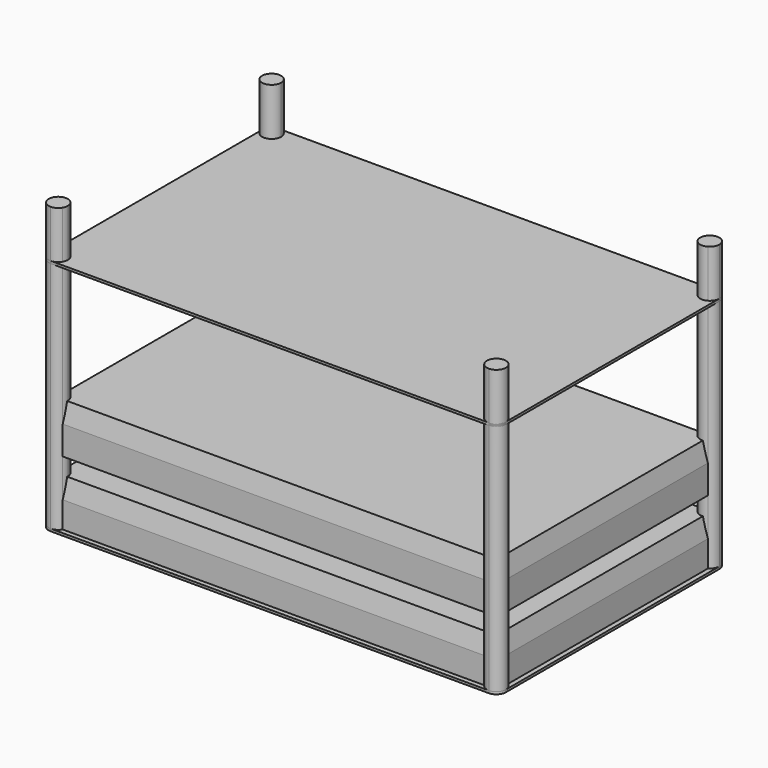
from build123d import *

# Parameters (mm, degrees)
F1_DEPTH = 6.35
F2_START = 6.35
F2_DEPTH = 120.65
F3_SIZE2 = 10.7978733328
F3_SIZE  = 50.8
F4_START = 6.35
F4_DEPTH = 755.65
F5_START = 628.65
F5_DEPTH = 6.35
F6_START = 177.8
F6_DEPTH = 127
F7_SIZE2 = 10.7978733328
F7_SIZE  = 50.8


# Not quite as in the source:
# - a feature names something its author has since deleted; it is built from what else it names


with BuildPart() as f1:
    # F0 (on Top) → F1 (new body)
    with BuildSketch(Plane.XY):
        Polygon((-421.6065403938, 372.1638967734), (-535.9065403938, 372.1638967734), (-535.9065403938, -364.4361032266), (-421.6065403938, -364.4361032266), (-383.5065403938, -364.4361032266), (378.4934596062, -364.4361032266), (416.5934596062, -364.4361032266), (530.8934596062, -364.4361032266), (530.8934596062, -219.4858193398), (530.8934596062, 237.7141806602), (530.8934596062, 372.1638967734), (416.5934596062, 372.1638967734), (378.4934596062, 372.1638967734), (-383.5065403938, 372.1638967734), align=None)
        Polygon((530.8934596062, 384.8638967734), (-535.9065403938, 384.8638967734), (-535.9065403938, 372.1638967734), (-421.6065403938, 372.1638967734), (-383.5065403938, 372.1638967734), (378.4934596062, 372.1638967734), (416.5934596062, 372.1638967734), (530.8934596062, 372.1638967734), align=None)
        Polygon((-421.6065403938, -364.4361032266), (-535.9065403938, -364.4361032266), (-535.9065403938, -377.1361032266), (530.8934596062, -377.1361032266), (530.8934596062, -364.4361032266), (416.5934596062, -364.4361032266), (378.4934596062, -364.4361032266), (-383.5065403938, -364.4361032266), align=None)
        with BuildLine():
            Line((607.0934596062, -351.7361032266), (607.0934596062, 359.4638967734))
            ThreePointArc((607.0934596062, 359.4638967734), (603.6905048623, 346.7638967734), (594.3934596062, 337.4668515172))
            Line((594.3934596062, 337.4668515172), (594.3934596062, 22.9138967734))
            Line((594.3934596062, 22.9138967734), (594.3934596062, -15.1861032266))
            Line((594.3934596062, -15.1861032266), (594.3934596062, -329.7390579705))
            ThreePointArc((594.3934596062, -329.7390579705), (603.6905048623, -339.0361032266), (607.0934596062, -351.7361032266))
        make_face()
        with BuildLine():
            ThreePointArc((-599.4065403938, 337.4668515172), (-608.70358565, 346.7638967734), (-612.1065403938, 359.4638967734))
            Line((-612.1065403938, 359.4638967734), (-612.1065403938, -351.7361032266))
            ThreePointArc((-612.1065403938, -351.7361032266), (-608.70358565, -339.0361032266), (-599.4065403938, -329.7390579705))
            Line((-599.4065403938, -329.7390579705), (-599.4065403938, -15.1861032266))
            Line((-599.4065403938, -15.1861032266), (-599.4065403938, 22.9138967734))
            Line((-599.4065403938, 22.9138967734), (-599.4065403938, 337.4668515172))
        make_face()
        with BuildLine():
            ThreePointArc((-561.3065403938, 359.4638967734), (-562.1720244061, 366.037900519), (-564.7094951377, 372.1638967734))
            Line((-564.7094951377, 372.1638967734), (-586.7065403938, 372.1638967734))
            ThreePointArc((-586.7065403938, 372.1638967734), (-595.6867965149, 368.4441528944), (-599.4065403938, 359.4638967734))
            Line((-599.4065403938, 359.4638967734), (-599.4065403938, 337.4668515172))
            ThreePointArc((-599.4065403938, 337.4668515172), (-574.0065403938, 337.4668515172), (-561.3065403938, 359.4638967734))
        make_face()
        with BuildLine():
            Line((581.6934596062, 372.1638967734), (559.69641435, 372.1638967734))
            ThreePointArc((559.69641435, 372.1638967734), (563.732947364, 341.5033845312), (594.3934596062, 337.4668515172))
            Line((594.3934596062, 337.4668515172), (594.3934596062, 359.4638967734))
            ThreePointArc((594.3934596062, 359.4638967734), (590.6737157272, 368.4441528944), (581.6934596062, 372.1638967734))
        make_face()
        with BuildLine():
            ThreePointArc((-561.3065403938, -351.7361032266), (-574.0065403938, -329.7390579705), (-599.4065403938, -329.7390579705))
            Line((-599.4065403938, -329.7390579705), (-599.4065403938, -351.7361032266))
            ThreePointArc((-599.4065403938, -351.7361032266), (-595.6867965149, -360.7163593477), (-586.7065403938, -364.4361032266))
            Line((-586.7065403938, -364.4361032266), (-564.7094951377, -364.4361032266))
            ThreePointArc((-564.7094951377, -364.4361032266), (-562.1720244061, -358.3101069722), (-561.3065403938, -351.7361032266))
        make_face()
        with BuildLine():
            Line((-535.9065403938, 372.1638967734), (-564.7094951377, 372.1638967734))
            ThreePointArc((-564.7094951377, 372.1638967734), (-562.1720244061, 366.037900519), (-561.3065403938, 359.4638967734))
            ThreePointArc((-561.3065403938, 359.4638967734), (-574.0065403938, 337.4668515172), (-599.4065403938, 337.4668515172))
            Line((-599.4065403938, 337.4668515172), (-599.4065403938, 22.9138967734))
            Line((-599.4065403938, 22.9138967734), (-599.4065403938, -15.1861032266))
            Line((-599.4065403938, -15.1861032266), (-599.4065403938, -329.7390579705))
            ThreePointArc((-599.4065403938, -329.7390579705), (-574.0065403938, -329.7390579705), (-561.3065403938, -351.7361032266))
            ThreePointArc((-561.3065403938, -351.7361032266), (-562.1720244061, -358.3101069722), (-564.7094951377, -364.4361032266))
            Line((-564.7094951377, -364.4361032266), (-535.9065403938, -364.4361032266))
            Line((-535.9065403938, -364.4361032266), (-535.9065403938, 372.1638967734))
        make_face()
        with BuildLine():
            Line((594.3934596062, -351.7361032266), (594.3934596062, -329.7390579705))
            ThreePointArc((594.3934596062, -329.7390579705), (563.732947364, -333.7755909845), (559.69641435, -364.4361032266))
            Line((559.69641435, -364.4361032266), (581.6934596062, -364.4361032266))
            ThreePointArc((581.6934596062, -364.4361032266), (590.6737157272, -360.7163593477), (594.3934596062, -351.7361032266))
        make_face()
        with BuildLine():
            Line((559.69641435, 372.1638967734), (530.8934596062, 372.1638967734))
            Line((530.8934596062, 372.1638967734), (530.8934596062, 237.7141806602))
            Line((530.8934596062, 237.7141806602), (530.8934596062, -219.4858193398))
            Line((530.8934596062, -219.4858193398), (530.8934596062, -364.4361032266))
            Line((530.8934596062, -364.4361032266), (559.69641435, -364.4361032266))
            ThreePointArc((559.69641435, -364.4361032266), (563.732947364, -333.7755909845), (594.3934596062, -329.7390579705))
            Line((594.3934596062, -329.7390579705), (594.3934596062, -15.1861032266))
            Line((594.3934596062, -15.1861032266), (594.3934596062, 22.9138967734))
            Line((594.3934596062, 22.9138967734), (594.3934596062, 337.4668515172))
            ThreePointArc((594.3934596062, 337.4668515172), (563.732947364, 341.5033845312), (559.69641435, 372.1638967734))
        make_face()
        with BuildLine():
            ThreePointArc((581.6934596062, -377.1361032266), (599.6539718483, -369.6966154688), (607.0934596062, -351.7361032266))
            ThreePointArc((607.0934596062, -351.7361032266), (603.6905048623, -339.0361032266), (594.3934596062, -329.7390579705))
            Line((594.3934596062, -329.7390579705), (594.3934596062, -351.7361032266))
            ThreePointArc((594.3934596062, -351.7361032266), (590.6737157272, -360.7163593477), (581.6934596062, -364.4361032266))
            Line((581.6934596062, -364.4361032266), (559.69641435, -364.4361032266))
            ThreePointArc((559.69641435, -364.4361032266), (568.9934596062, -373.7331484828), (581.6934596062, -377.1361032266))
        make_face()
        with BuildLine():
            Line((530.8934596062, -364.4361032266), (530.8934596062, -377.1361032266))
            Line((530.8934596062, -377.1361032266), (581.6934596062, -377.1361032266))
            ThreePointArc((581.6934596062, -377.1361032266), (568.9934596062, -373.7331484828), (559.69641435, -364.4361032266))
            Line((559.69641435, -364.4361032266), (530.8934596062, -364.4361032266))
        make_face()
        with BuildLine():
            ThreePointArc((607.0934596062, 359.4638967734), (599.6539718483, 377.4244090155), (581.6934596062, 384.8638967734))
            ThreePointArc((581.6934596062, 384.8638967734), (568.9934596062, 381.4609420295), (559.69641435, 372.1638967734))
            Line((559.69641435, 372.1638967734), (581.6934596062, 372.1638967734))
            ThreePointArc((581.6934596062, 372.1638967734), (590.6737157272, 368.4441528944), (594.3934596062, 359.4638967734))
            Line((594.3934596062, 359.4638967734), (594.3934596062, 337.4668515172))
            ThreePointArc((594.3934596062, 337.4668515172), (603.6905048623, 346.7638967734), (607.0934596062, 359.4638967734))
        make_face()
        with BuildLine():
            Line((581.6934596062, 384.8638967734), (530.8934596062, 384.8638967734))
            Line((530.8934596062, 384.8638967734), (530.8934596062, 372.1638967734))
            Line((530.8934596062, 372.1638967734), (559.69641435, 372.1638967734))
            ThreePointArc((559.69641435, 372.1638967734), (568.9934596062, 381.4609420295), (581.6934596062, 384.8638967734))
        make_face()
        with BuildLine():
            Line((-535.9065403938, -377.1361032266), (-535.9065403938, -364.4361032266))
            Line((-535.9065403938, -364.4361032266), (-564.7094951377, -364.4361032266))
            ThreePointArc((-564.7094951377, -364.4361032266), (-574.0065403938, -373.7331484828), (-586.7065403938, -377.1361032266))
            Line((-586.7065403938, -377.1361032266), (-535.9065403938, -377.1361032266))
        make_face()
        with BuildLine():
            ThreePointArc((-599.4065403938, -329.7390579705), (-608.70358565, -339.0361032266), (-612.1065403938, -351.7361032266))
            ThreePointArc((-612.1065403938, -351.7361032266), (-604.667052636, -369.6966154688), (-586.7065403938, -377.1361032266))
            ThreePointArc((-586.7065403938, -377.1361032266), (-574.0065403938, -373.7331484828), (-564.7094951377, -364.4361032266))
            Line((-564.7094951377, -364.4361032266), (-586.7065403938, -364.4361032266))
            ThreePointArc((-586.7065403938, -364.4361032266), (-595.6867965149, -360.7163593477), (-599.4065403938, -351.7361032266))
            Line((-599.4065403938, -351.7361032266), (-599.4065403938, -329.7390579705))
        make_face()
        with BuildLine():
            Line((-535.9065403938, 384.8638967734), (-586.7065403938, 384.8638967734))
            ThreePointArc((-586.7065403938, 384.8638967734), (-574.0065403938, 381.4609420295), (-564.7094951377, 372.1638967734))
            Line((-564.7094951377, 372.1638967734), (-535.9065403938, 372.1638967734))
            Line((-535.9065403938, 372.1638967734), (-535.9065403938, 384.8638967734))
        make_face()
        with BuildLine():
            ThreePointArc((-564.7094951377, 372.1638967734), (-574.0065403938, 381.4609420295), (-586.7065403938, 384.8638967734))
            ThreePointArc((-586.7065403938, 384.8638967734), (-604.667052636, 377.4244090155), (-612.1065403938, 359.4638967734))
            ThreePointArc((-612.1065403938, 359.4638967734), (-608.70358565, 346.7638967734), (-599.4065403938, 337.4668515172))
            Line((-599.4065403938, 337.4668515172), (-599.4065403938, 359.4638967734))
            ThreePointArc((-599.4065403938, 359.4638967734), (-595.6867965149, 368.4441528944), (-586.7065403938, 372.1638967734))
            Line((-586.7065403938, 372.1638967734), (-564.7094951377, 372.1638967734))
        make_face()
    extrude(amount=F1_DEPTH)


with BuildPart() as f2:
    # F0 (on Top) → F2 (new body)
    with BuildSketch(Plane.XY.offset(F2_START)):
        Polygon((-421.6065403938, 372.1638967734), (-535.9065403938, 372.1638967734), (-535.9065403938, -364.4361032266), (-421.6065403938, -364.4361032266), (-383.5065403938, -364.4361032266), (378.4934596062, -364.4361032266), (416.5934596062, -364.4361032266), (530.8934596062, -364.4361032266), (530.8934596062, -219.4858193398), (530.8934596062, 237.7141806602), (530.8934596062, 372.1638967734), (416.5934596062, 372.1638967734), (378.4934596062, 372.1638967734), (-383.5065403938, 372.1638967734), align=None)
        with BuildLine():
            Line((-535.9065403938, 372.1638967734), (-564.7094951377, 372.1638967734))
            ThreePointArc((-564.7094951377, 372.1638967734), (-562.1720244061, 366.037900519), (-561.3065403938, 359.4638967734))
            ThreePointArc((-561.3065403938, 359.4638967734), (-574.0065403938, 337.4668515172), (-599.4065403938, 337.4668515172))
            Line((-599.4065403938, 337.4668515172), (-599.4065403938, 22.9138967734))
            Line((-599.4065403938, 22.9138967734), (-599.4065403938, -15.1861032266))
            Line((-599.4065403938, -15.1861032266), (-599.4065403938, -329.7390579705))
            ThreePointArc((-599.4065403938, -329.7390579705), (-574.0065403938, -329.7390579705), (-561.3065403938, -351.7361032266))
            ThreePointArc((-561.3065403938, -351.7361032266), (-562.1720244061, -358.3101069722), (-564.7094951377, -364.4361032266))
            Line((-564.7094951377, -364.4361032266), (-535.9065403938, -364.4361032266))
            Line((-535.9065403938, -364.4361032266), (-535.9065403938, 372.1638967734))
        make_face()
        with BuildLine():
            Line((559.69641435, 372.1638967734), (530.8934596062, 372.1638967734))
            Line((530.8934596062, 372.1638967734), (530.8934596062, 237.7141806602))
            Line((530.8934596062, 237.7141806602), (530.8934596062, -219.4858193398))
            Line((530.8934596062, -219.4858193398), (530.8934596062, -364.4361032266))
            Line((530.8934596062, -364.4361032266), (559.69641435, -364.4361032266))
            ThreePointArc((559.69641435, -364.4361032266), (563.732947364, -333.7755909845), (594.3934596062, -329.7390579705))
            Line((594.3934596062, -329.7390579705), (594.3934596062, -15.1861032266))
            Line((594.3934596062, -15.1861032266), (594.3934596062, 22.9138967734))
            Line((594.3934596062, 22.9138967734), (594.3934596062, 337.4668515172))
            ThreePointArc((594.3934596062, 337.4668515172), (563.732947364, 341.5033845312), (559.69641435, 372.1638967734))
        make_face()
        with BuildLine():
            ThreePointArc((-561.3065403938, 359.4638967734), (-562.1720244061, 366.037900519), (-564.7094951377, 372.1638967734))
            Line((-564.7094951377, 372.1638967734), (-586.7065403938, 372.1638967734))
            ThreePointArc((-586.7065403938, 372.1638967734), (-595.6867965149, 368.4441528944), (-599.4065403938, 359.4638967734))
            Line((-599.4065403938, 359.4638967734), (-599.4065403938, 337.4668515172))
            ThreePointArc((-599.4065403938, 337.4668515172), (-574.0065403938, 337.4668515172), (-561.3065403938, 359.4638967734))
        make_face()
        with BuildLine():
            Line((581.6934596062, 372.1638967734), (559.69641435, 372.1638967734))
            ThreePointArc((559.69641435, 372.1638967734), (563.732947364, 341.5033845312), (594.3934596062, 337.4668515172))
            Line((594.3934596062, 337.4668515172), (594.3934596062, 359.4638967734))
            ThreePointArc((594.3934596062, 359.4638967734), (590.6737157272, 368.4441528944), (581.6934596062, 372.1638967734))
        make_face()
        with BuildLine():
            ThreePointArc((-561.3065403938, -351.7361032266), (-574.0065403938, -329.7390579705), (-599.4065403938, -329.7390579705))
            Line((-599.4065403938, -329.7390579705), (-599.4065403938, -351.7361032266))
            ThreePointArc((-599.4065403938, -351.7361032266), (-595.6867965149, -360.7163593477), (-586.7065403938, -364.4361032266))
            Line((-586.7065403938, -364.4361032266), (-564.7094951377, -364.4361032266))
            ThreePointArc((-564.7094951377, -364.4361032266), (-562.1720244061, -358.3101069722), (-561.3065403938, -351.7361032266))
        make_face()
        with BuildLine():
            Line((594.3934596062, -351.7361032266), (594.3934596062, -329.7390579705))
            ThreePointArc((594.3934596062, -329.7390579705), (563.732947364, -333.7755909845), (559.69641435, -364.4361032266))
            Line((559.69641435, -364.4361032266), (581.6934596062, -364.4361032266))
            ThreePointArc((581.6934596062, -364.4361032266), (590.6737157272, -360.7163593477), (594.3934596062, -351.7361032266))
        make_face()
    extrude(amount=F2_DEPTH)

    # F3
    f3_edges = [f2.edges().sort_by_distance(p)[0] for p in [
        (590.673716, 368.444153, 127),
        (-2.50654, 372.163897, 127),
        (-595.686797, 368.444153, 127),
        (-599.40654, 3.863897, 127),
        (-595.686797, -360.716359, 127),
        (-2.50654, -364.436103, 127),
        (590.673716, -360.716359, 127),
        (594.39346, 3.863897, 127),
    ]]
    chamfer(f3_edges, length=F3_SIZE, length2=F3_SIZE2)


with BuildPart() as f4:
    # F0 (on Top) → F4 (new body)
    with BuildSketch(Plane.XY.offset(F4_START)):
        with BuildLine():
            ThreePointArc((581.6934596062, -377.1361032266), (599.6539718483, -369.6966154688), (607.0934596062, -351.7361032266))
            ThreePointArc((607.0934596062, -351.7361032266), (603.6905048623, -339.0361032266), (594.3934596062, -329.7390579705))
            Line((594.3934596062, -329.7390579705), (594.3934596062, -351.7361032266))
            ThreePointArc((594.3934596062, -351.7361032266), (590.6737157272, -360.7163593477), (581.6934596062, -364.4361032266))
            Line((581.6934596062, -364.4361032266), (559.69641435, -364.4361032266))
            ThreePointArc((559.69641435, -364.4361032266), (568.9934596062, -373.7331484828), (581.6934596062, -377.1361032266))
        make_face()
        with BuildLine():
            Line((594.3934596062, -351.7361032266), (594.3934596062, -329.7390579705))
            ThreePointArc((594.3934596062, -329.7390579705), (563.732947364, -333.7755909845), (559.69641435, -364.4361032266))
            Line((559.69641435, -364.4361032266), (581.6934596062, -364.4361032266))
            ThreePointArc((581.6934596062, -364.4361032266), (590.6737157272, -360.7163593477), (594.3934596062, -351.7361032266))
        make_face()
    extrude(amount=F4_DEPTH)


with BuildPart() as f4b:
    # F0 (on Top) → F4, piece 2 (new body)
    with BuildSketch(Plane.XY.offset(F4_START)):
        with BuildLine():
            ThreePointArc((-561.3065403938, 359.4638967734), (-562.1720244061, 366.037900519), (-564.7094951377, 372.1638967734))
            Line((-564.7094951377, 372.1638967734), (-586.7065403938, 372.1638967734))
            ThreePointArc((-586.7065403938, 372.1638967734), (-595.6867965149, 368.4441528944), (-599.4065403938, 359.4638967734))
            Line((-599.4065403938, 359.4638967734), (-599.4065403938, 337.4668515172))
            ThreePointArc((-599.4065403938, 337.4668515172), (-574.0065403938, 337.4668515172), (-561.3065403938, 359.4638967734))
        make_face()
        with BuildLine():
            ThreePointArc((-564.7094951377, 372.1638967734), (-574.0065403938, 381.4609420295), (-586.7065403938, 384.8638967734))
            ThreePointArc((-586.7065403938, 384.8638967734), (-604.667052636, 377.4244090155), (-612.1065403938, 359.4638967734))
            ThreePointArc((-612.1065403938, 359.4638967734), (-608.70358565, 346.7638967734), (-599.4065403938, 337.4668515172))
            Line((-599.4065403938, 337.4668515172), (-599.4065403938, 359.4638967734))
            ThreePointArc((-599.4065403938, 359.4638967734), (-595.6867965149, 368.4441528944), (-586.7065403938, 372.1638967734))
            Line((-586.7065403938, 372.1638967734), (-564.7094951377, 372.1638967734))
        make_face()
    extrude(amount=F4_DEPTH)


with BuildPart() as f4c:
    # F0 (on Top) → F4, piece 3 (new body)
    with BuildSketch(Plane.XY.offset(F4_START)):
        with BuildLine():
            ThreePointArc((-561.3065403938, -351.7361032266), (-574.0065403938, -329.7390579705), (-599.4065403938, -329.7390579705))
            Line((-599.4065403938, -329.7390579705), (-599.4065403938, -351.7361032266))
            ThreePointArc((-599.4065403938, -351.7361032266), (-595.6867965149, -360.7163593477), (-586.7065403938, -364.4361032266))
            Line((-586.7065403938, -364.4361032266), (-564.7094951377, -364.4361032266))
            ThreePointArc((-564.7094951377, -364.4361032266), (-562.1720244061, -358.3101069722), (-561.3065403938, -351.7361032266))
        make_face()
        with BuildLine():
            ThreePointArc((-599.4065403938, -329.7390579705), (-608.70358565, -339.0361032266), (-612.1065403938, -351.7361032266))
            ThreePointArc((-612.1065403938, -351.7361032266), (-604.667052636, -369.6966154688), (-586.7065403938, -377.1361032266))
            ThreePointArc((-586.7065403938, -377.1361032266), (-574.0065403938, -373.7331484828), (-564.7094951377, -364.4361032266))
            Line((-564.7094951377, -364.4361032266), (-586.7065403938, -364.4361032266))
            ThreePointArc((-586.7065403938, -364.4361032266), (-595.6867965149, -360.7163593477), (-599.4065403938, -351.7361032266))
            Line((-599.4065403938, -351.7361032266), (-599.4065403938, -329.7390579705))
        make_face()
    extrude(amount=F4_DEPTH)


with BuildPart() as f4d:
    # F0 (on Top) → F4, piece 4 (new body)
    with BuildSketch(Plane.XY.offset(F4_START)):
        with BuildLine():
            ThreePointArc((607.0934596062, 359.4638967734), (599.6539718483, 377.4244090155), (581.6934596062, 384.8638967734))
            ThreePointArc((581.6934596062, 384.8638967734), (568.9934596062, 381.4609420295), (559.69641435, 372.1638967734))
            Line((559.69641435, 372.1638967734), (581.6934596062, 372.1638967734))
            ThreePointArc((581.6934596062, 372.1638967734), (590.6737157272, 368.4441528944), (594.3934596062, 359.4638967734))
            Line((594.3934596062, 359.4638967734), (594.3934596062, 337.4668515172))
            ThreePointArc((594.3934596062, 337.4668515172), (603.6905048623, 346.7638967734), (607.0934596062, 359.4638967734))
        make_face()
        with BuildLine():
            Line((581.6934596062, 372.1638967734), (559.69641435, 372.1638967734))
            ThreePointArc((559.69641435, 372.1638967734), (563.732947364, 341.5033845312), (594.3934596062, 337.4668515172))
            Line((594.3934596062, 337.4668515172), (594.3934596062, 359.4638967734))
            ThreePointArc((594.3934596062, 359.4638967734), (590.6737157272, 368.4441528944), (581.6934596062, 372.1638967734))
        make_face()
    extrude(amount=F4_DEPTH)


with BuildPart() as f5:
    # F0 (on Top) → F5 (new body)
    with BuildSketch(Plane.XY.offset(F5_START)):
        with BuildLine():
            ThreePointArc((-599.4065403938, 337.4668515172), (-608.70358565, 346.7638967734), (-612.1065403938, 359.4638967734))
            Line((-612.1065403938, 359.4638967734), (-612.1065403938, -351.7361032266))
            ThreePointArc((-612.1065403938, -351.7361032266), (-608.70358565, -339.0361032266), (-599.4065403938, -329.7390579705))
            Line((-599.4065403938, -329.7390579705), (-599.4065403938, -15.1861032266))
            Line((-599.4065403938, -15.1861032266), (-599.4065403938, 22.9138967734))
            Line((-599.4065403938, 22.9138967734), (-599.4065403938, 337.4668515172))
        make_face()
        with BuildLine():
            Line((-535.9065403938, 372.1638967734), (-564.7094951377, 372.1638967734))
            ThreePointArc((-564.7094951377, 372.1638967734), (-562.1720244061, 366.037900519), (-561.3065403938, 359.4638967734))
            ThreePointArc((-561.3065403938, 359.4638967734), (-574.0065403938, 337.4668515172), (-599.4065403938, 337.4668515172))
            Line((-599.4065403938, 337.4668515172), (-599.4065403938, 22.9138967734))
            Line((-599.4065403938, 22.9138967734), (-599.4065403938, -15.1861032266))
            Line((-599.4065403938, -15.1861032266), (-599.4065403938, -329.7390579705))
            ThreePointArc((-599.4065403938, -329.7390579705), (-574.0065403938, -329.7390579705), (-561.3065403938, -351.7361032266))
            ThreePointArc((-561.3065403938, -351.7361032266), (-562.1720244061, -358.3101069722), (-564.7094951377, -364.4361032266))
            Line((-564.7094951377, -364.4361032266), (-535.9065403938, -364.4361032266))
            Line((-535.9065403938, -364.4361032266), (-535.9065403938, 372.1638967734))
        make_face()
        with BuildLine():
            ThreePointArc((-561.3065403938, 359.4638967734), (-562.1720244061, 366.037900519), (-564.7094951377, 372.1638967734))
            Line((-564.7094951377, 372.1638967734), (-586.7065403938, 372.1638967734))
            ThreePointArc((-586.7065403938, 372.1638967734), (-595.6867965149, 368.4441528944), (-599.4065403938, 359.4638967734))
            Line((-599.4065403938, 359.4638967734), (-599.4065403938, 337.4668515172))
            ThreePointArc((-599.4065403938, 337.4668515172), (-574.0065403938, 337.4668515172), (-561.3065403938, 359.4638967734))
        make_face()
        with BuildLine():
            ThreePointArc((-564.7094951377, 372.1638967734), (-574.0065403938, 381.4609420295), (-586.7065403938, 384.8638967734))
            ThreePointArc((-586.7065403938, 384.8638967734), (-604.667052636, 377.4244090155), (-612.1065403938, 359.4638967734))
            ThreePointArc((-612.1065403938, 359.4638967734), (-608.70358565, 346.7638967734), (-599.4065403938, 337.4668515172))
            Line((-599.4065403938, 337.4668515172), (-599.4065403938, 359.4638967734))
            ThreePointArc((-599.4065403938, 359.4638967734), (-595.6867965149, 368.4441528944), (-586.7065403938, 372.1638967734))
            Line((-586.7065403938, 372.1638967734), (-564.7094951377, 372.1638967734))
        make_face()
        Polygon((-421.6065403938, 372.1638967734), (-535.9065403938, 372.1638967734), (-535.9065403938, -364.4361032266), (-421.6065403938, -364.4361032266), (-383.5065403938, -364.4361032266), (378.4934596062, -364.4361032266), (416.5934596062, -364.4361032266), (530.8934596062, -364.4361032266), (530.8934596062, -219.4858193398), (530.8934596062, 237.7141806602), (530.8934596062, 372.1638967734), (416.5934596062, 372.1638967734), (378.4934596062, 372.1638967734), (-383.5065403938, 372.1638967734), align=None)
        with BuildLine():
            Line((-535.9065403938, 384.8638967734), (-586.7065403938, 384.8638967734))
            ThreePointArc((-586.7065403938, 384.8638967734), (-574.0065403938, 381.4609420295), (-564.7094951377, 372.1638967734))
            Line((-564.7094951377, 372.1638967734), (-535.9065403938, 372.1638967734))
            Line((-535.9065403938, 372.1638967734), (-535.9065403938, 384.8638967734))
        make_face()
        Polygon((530.8934596062, 384.8638967734), (-535.9065403938, 384.8638967734), (-535.9065403938, 372.1638967734), (-421.6065403938, 372.1638967734), (-383.5065403938, 372.1638967734), (378.4934596062, 372.1638967734), (416.5934596062, 372.1638967734), (530.8934596062, 372.1638967734), align=None)
        with BuildLine():
            ThreePointArc((-599.4065403938, -329.7390579705), (-608.70358565, -339.0361032266), (-612.1065403938, -351.7361032266))
            ThreePointArc((-612.1065403938, -351.7361032266), (-604.667052636, -369.6966154688), (-586.7065403938, -377.1361032266))
            ThreePointArc((-586.7065403938, -377.1361032266), (-574.0065403938, -373.7331484828), (-564.7094951377, -364.4361032266))
            Line((-564.7094951377, -364.4361032266), (-586.7065403938, -364.4361032266))
            ThreePointArc((-586.7065403938, -364.4361032266), (-595.6867965149, -360.7163593477), (-599.4065403938, -351.7361032266))
            Line((-599.4065403938, -351.7361032266), (-599.4065403938, -329.7390579705))
        make_face()
        with BuildLine():
            ThreePointArc((-561.3065403938, -351.7361032266), (-574.0065403938, -329.7390579705), (-599.4065403938, -329.7390579705))
            Line((-599.4065403938, -329.7390579705), (-599.4065403938, -351.7361032266))
            ThreePointArc((-599.4065403938, -351.7361032266), (-595.6867965149, -360.7163593477), (-586.7065403938, -364.4361032266))
            Line((-586.7065403938, -364.4361032266), (-564.7094951377, -364.4361032266))
            ThreePointArc((-564.7094951377, -364.4361032266), (-562.1720244061, -358.3101069722), (-561.3065403938, -351.7361032266))
        make_face()
        with BuildLine():
            Line((-535.9065403938, -377.1361032266), (-535.9065403938, -364.4361032266))
            Line((-535.9065403938, -364.4361032266), (-564.7094951377, -364.4361032266))
            ThreePointArc((-564.7094951377, -364.4361032266), (-574.0065403938, -373.7331484828), (-586.7065403938, -377.1361032266))
            Line((-586.7065403938, -377.1361032266), (-535.9065403938, -377.1361032266))
        make_face()
        Polygon((-421.6065403938, -364.4361032266), (-535.9065403938, -364.4361032266), (-535.9065403938, -377.1361032266), (530.8934596062, -377.1361032266), (530.8934596062, -364.4361032266), (416.5934596062, -364.4361032266), (378.4934596062, -364.4361032266), (-383.5065403938, -364.4361032266), align=None)
        with BuildLine():
            Line((581.6934596062, 384.8638967734), (530.8934596062, 384.8638967734))
            Line((530.8934596062, 384.8638967734), (530.8934596062, 372.1638967734))
            Line((530.8934596062, 372.1638967734), (559.69641435, 372.1638967734))
            ThreePointArc((559.69641435, 372.1638967734), (568.9934596062, 381.4609420295), (581.6934596062, 384.8638967734))
        make_face()
        with BuildLine():
            Line((581.6934596062, 372.1638967734), (559.69641435, 372.1638967734))
            ThreePointArc((559.69641435, 372.1638967734), (563.732947364, 341.5033845312), (594.3934596062, 337.4668515172))
            Line((594.3934596062, 337.4668515172), (594.3934596062, 359.4638967734))
            ThreePointArc((594.3934596062, 359.4638967734), (590.6737157272, 368.4441528944), (581.6934596062, 372.1638967734))
        make_face()
        with BuildLine():
            Line((559.69641435, 372.1638967734), (530.8934596062, 372.1638967734))
            Line((530.8934596062, 372.1638967734), (530.8934596062, 237.7141806602))
            Line((530.8934596062, 237.7141806602), (530.8934596062, -219.4858193398))
            Line((530.8934596062, -219.4858193398), (530.8934596062, -364.4361032266))
            Line((530.8934596062, -364.4361032266), (559.69641435, -364.4361032266))
            ThreePointArc((559.69641435, -364.4361032266), (563.732947364, -333.7755909845), (594.3934596062, -329.7390579705))
            Line((594.3934596062, -329.7390579705), (594.3934596062, -15.1861032266))
            Line((594.3934596062, -15.1861032266), (594.3934596062, 22.9138967734))
            Line((594.3934596062, 22.9138967734), (594.3934596062, 337.4668515172))
            ThreePointArc((594.3934596062, 337.4668515172), (563.732947364, 341.5033845312), (559.69641435, 372.1638967734))
        make_face()
        with BuildLine():
            Line((607.0934596062, -351.7361032266), (607.0934596062, 359.4638967734))
            ThreePointArc((607.0934596062, 359.4638967734), (603.6905048623, 346.7638967734), (594.3934596062, 337.4668515172))
            Line((594.3934596062, 337.4668515172), (594.3934596062, 22.9138967734))
            Line((594.3934596062, 22.9138967734), (594.3934596062, -15.1861032266))
            Line((594.3934596062, -15.1861032266), (594.3934596062, -329.7390579705))
            ThreePointArc((594.3934596062, -329.7390579705), (603.6905048623, -339.0361032266), (607.0934596062, -351.7361032266))
        make_face()
        with BuildLine():
            ThreePointArc((607.0934596062, 359.4638967734), (599.6539718483, 377.4244090155), (581.6934596062, 384.8638967734))
            ThreePointArc((581.6934596062, 384.8638967734), (568.9934596062, 381.4609420295), (559.69641435, 372.1638967734))
            Line((559.69641435, 372.1638967734), (581.6934596062, 372.1638967734))
            ThreePointArc((581.6934596062, 372.1638967734), (590.6737157272, 368.4441528944), (594.3934596062, 359.4638967734))
            Line((594.3934596062, 359.4638967734), (594.3934596062, 337.4668515172))
            ThreePointArc((594.3934596062, 337.4668515172), (603.6905048623, 346.7638967734), (607.0934596062, 359.4638967734))
        make_face()
        with BuildLine():
            Line((530.8934596062, -364.4361032266), (530.8934596062, -377.1361032266))
            Line((530.8934596062, -377.1361032266), (581.6934596062, -377.1361032266))
            ThreePointArc((581.6934596062, -377.1361032266), (568.9934596062, -373.7331484828), (559.69641435, -364.4361032266))
            Line((559.69641435, -364.4361032266), (530.8934596062, -364.4361032266))
        make_face()
        with BuildLine():
            Line((594.3934596062, -351.7361032266), (594.3934596062, -329.7390579705))
            ThreePointArc((594.3934596062, -329.7390579705), (563.732947364, -333.7755909845), (559.69641435, -364.4361032266))
            Line((559.69641435, -364.4361032266), (581.6934596062, -364.4361032266))
            ThreePointArc((581.6934596062, -364.4361032266), (590.6737157272, -360.7163593477), (594.3934596062, -351.7361032266))
        make_face()
        with BuildLine():
            ThreePointArc((581.6934596062, -377.1361032266), (599.6539718483, -369.6966154688), (607.0934596062, -351.7361032266))
            ThreePointArc((607.0934596062, -351.7361032266), (603.6905048623, -339.0361032266), (594.3934596062, -329.7390579705))
            Line((594.3934596062, -329.7390579705), (594.3934596062, -351.7361032266))
            ThreePointArc((594.3934596062, -351.7361032266), (590.6737157272, -360.7163593477), (581.6934596062, -364.4361032266))
            Line((581.6934596062, -364.4361032266), (559.69641435, -364.4361032266))
            ThreePointArc((559.69641435, -364.4361032266), (568.9934596062, -373.7331484828), (581.6934596062, -377.1361032266))
        make_face()
    extrude(amount=F5_DEPTH)


with BuildPart() as f6:
    # F0 (on Top) → F6 (new body)
    with BuildSketch(Plane.XY.offset(F6_START)):
        with BuildLine():
            ThreePointArc((-561.3065403938, 359.4638967734), (-562.1720244061, 366.037900519), (-564.7094951377, 372.1638967734))
            Line((-564.7094951377, 372.1638967734), (-586.7065403938, 372.1638967734))
            ThreePointArc((-586.7065403938, 372.1638967734), (-595.6867965149, 368.4441528944), (-599.4065403938, 359.4638967734))
            Line((-599.4065403938, 359.4638967734), (-599.4065403938, 337.4668515172))
            ThreePointArc((-599.4065403938, 337.4668515172), (-574.0065403938, 337.4668515172), (-561.3065403938, 359.4638967734))
        make_face()
        with BuildLine():
            Line((-535.9065403938, 372.1638967734), (-564.7094951377, 372.1638967734))
            ThreePointArc((-564.7094951377, 372.1638967734), (-562.1720244061, 366.037900519), (-561.3065403938, 359.4638967734))
            ThreePointArc((-561.3065403938, 359.4638967734), (-574.0065403938, 337.4668515172), (-599.4065403938, 337.4668515172))
            Line((-599.4065403938, 337.4668515172), (-599.4065403938, 22.9138967734))
            Line((-599.4065403938, 22.9138967734), (-599.4065403938, -15.1861032266))
            Line((-599.4065403938, -15.1861032266), (-599.4065403938, -329.7390579705))
            ThreePointArc((-599.4065403938, -329.7390579705), (-574.0065403938, -329.7390579705), (-561.3065403938, -351.7361032266))
            ThreePointArc((-561.3065403938, -351.7361032266), (-562.1720244061, -358.3101069722), (-564.7094951377, -364.4361032266))
            Line((-564.7094951377, -364.4361032266), (-535.9065403938, -364.4361032266))
            Line((-535.9065403938, -364.4361032266), (-535.9065403938, 372.1638967734))
        make_face()
        Polygon((-421.6065403938, 372.1638967734), (-535.9065403938, 372.1638967734), (-535.9065403938, -364.4361032266), (-421.6065403938, -364.4361032266), (-383.5065403938, -364.4361032266), (378.4934596062, -364.4361032266), (416.5934596062, -364.4361032266), (530.8934596062, -364.4361032266), (530.8934596062, -219.4858193398), (530.8934596062, 237.7141806602), (530.8934596062, 372.1638967734), (416.5934596062, 372.1638967734), (378.4934596062, 372.1638967734), (-383.5065403938, 372.1638967734), align=None)
        with BuildLine():
            ThreePointArc((-561.3065403938, -351.7361032266), (-574.0065403938, -329.7390579705), (-599.4065403938, -329.7390579705))
            Line((-599.4065403938, -329.7390579705), (-599.4065403938, -351.7361032266))
            ThreePointArc((-599.4065403938, -351.7361032266), (-595.6867965149, -360.7163593477), (-586.7065403938, -364.4361032266))
            Line((-586.7065403938, -364.4361032266), (-564.7094951377, -364.4361032266))
            ThreePointArc((-564.7094951377, -364.4361032266), (-562.1720244061, -358.3101069722), (-561.3065403938, -351.7361032266))
        make_face()
        with BuildLine():
            Line((581.6934596062, 372.1638967734), (559.69641435, 372.1638967734))
            ThreePointArc((559.69641435, 372.1638967734), (563.732947364, 341.5033845312), (594.3934596062, 337.4668515172))
            Line((594.3934596062, 337.4668515172), (594.3934596062, 359.4638967734))
            ThreePointArc((594.3934596062, 359.4638967734), (590.6737157272, 368.4441528944), (581.6934596062, 372.1638967734))
        make_face()
        with BuildLine():
            Line((559.69641435, 372.1638967734), (530.8934596062, 372.1638967734))
            Line((530.8934596062, 372.1638967734), (530.8934596062, 237.7141806602))
            Line((530.8934596062, 237.7141806602), (530.8934596062, -219.4858193398))
            Line((530.8934596062, -219.4858193398), (530.8934596062, -364.4361032266))
            Line((530.8934596062, -364.4361032266), (559.69641435, -364.4361032266))
            ThreePointArc((559.69641435, -364.4361032266), (563.732947364, -333.7755909845), (594.3934596062, -329.7390579705))
            Line((594.3934596062, -329.7390579705), (594.3934596062, -15.1861032266))
            Line((594.3934596062, -15.1861032266), (594.3934596062, 22.9138967734))
            Line((594.3934596062, 22.9138967734), (594.3934596062, 337.4668515172))
            ThreePointArc((594.3934596062, 337.4668515172), (563.732947364, 341.5033845312), (559.69641435, 372.1638967734))
        make_face()
        with BuildLine():
            Line((594.3934596062, -351.7361032266), (594.3934596062, -329.7390579705))
            ThreePointArc((594.3934596062, -329.7390579705), (563.732947364, -333.7755909845), (559.69641435, -364.4361032266))
            Line((559.69641435, -364.4361032266), (581.6934596062, -364.4361032266))
            ThreePointArc((581.6934596062, -364.4361032266), (590.6737157272, -360.7163593477), (594.3934596062, -351.7361032266))
        make_face()
    extrude(amount=F6_DEPTH)

    # F7
    f7_edges = [f6.edges().sort_by_distance(p)[0] for p in [
        (-595.686797, 368.444153, 304.8),
        (-599.40654, 3.863897, 304.8),
        (-595.686797, -360.716359, 304.8),
        (-2.50654, -364.436103, 304.8),
        (590.673716, -360.716359, 304.8),
        (594.39346, 3.863897, 304.8),
        (590.673716, 368.444153, 304.8),
        (-2.50654, 372.163897, 304.8),
    ]]
    chamfer(f7_edges, length=F7_SIZE, length2=F7_SIZE2)


solid = Compound([f1.part, f2.part, f4.part, f4b.part, f4c.part, f4d.part, f5.part, f6.part])
